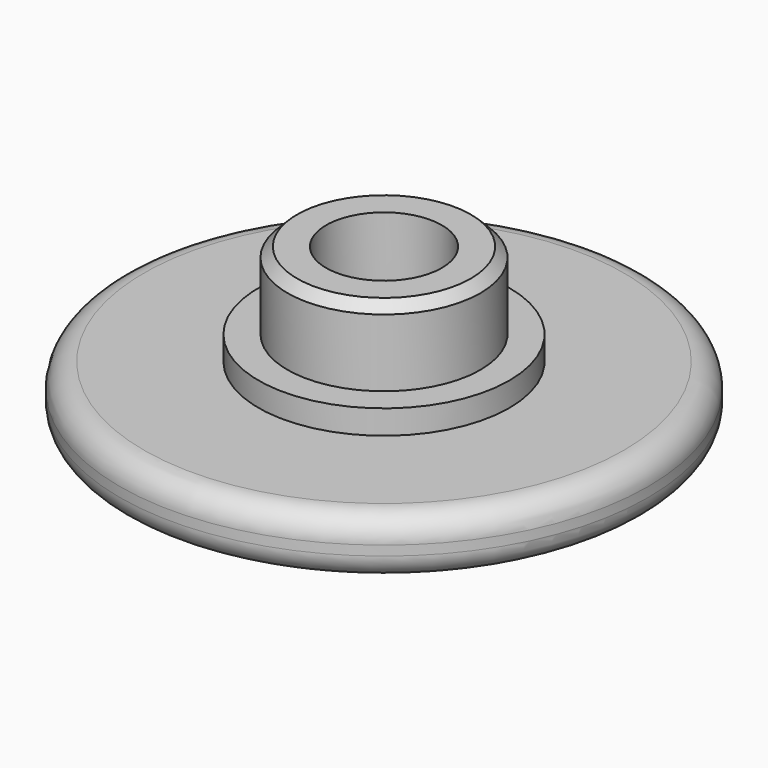
from build123d import *

# Parameters (mm, degrees)
F0_R      = 10.95
F1_DEPTH  = 2.4
F2_R      = 4
F3_DEPTH  = 4.2
F4_R      = 1
F5_R      = 5.2
F5_R_2    = 4
F6_DEPTH  = 1
F7_R      = 1
F8_R      = 8.5
F9_DEPTH  = 2
F11_SIZE  = 0.4
F12_R     = 3
F13_R     = 2.4
F14_DEPTH = 2.5


# Not quite as in the source:
# - a fillet or chamfer that OpenCascade refuses, or shapes differently, is made with other operations: its cross-section is extruded or revolved along the edge and cut away or added


with BuildPart() as f1:
    # F0 (on Top) → F1 (new body)
    with BuildSketch(Plane.XY):
        Circle(F0_R)
    extrude(amount=F1_DEPTH)

    # F2 (on face) → F3 (join)
    with BuildSketch(Plane.XY.offset(2.4)):
        Circle(F2_R)
    extrude(amount=F3_DEPTH)

    # F4
    f4_edges = [f1.edges().sort_by_distance(p)[0] for p in [
        (-10.95, 0, 2.4),
    ]]
    fillet(f4_edges, radius=F4_R)

    # F5 (on face) → F6 (join)
    with BuildSketch(Plane.XY.offset(2.4)):
        Circle(F5_R)
        Circle(F5_R_2, mode=Mode.SUBTRACT)
    extrude(amount=F6_DEPTH)

    # F7
    f7_edges = [f1.edges().sort_by_distance(p)[0] for p in [
        (-10.95, 0, 0),
    ]]
    fillet(f7_edges, radius=F7_R)

    # F8 (on face) → F9 (cut)
    with BuildSketch(Plane(origin=(0, 0, 0), x_dir=(1, 0, 0), z_dir=(0, 0, -1))):
        Circle(F8_R)
    extrude(amount=-F9_DEPTH, mode=Mode.SUBTRACT)

    # F10: fillet of radius 9 on 1 edges, made by hand

    # F10_s1 → F10_t2 (revolve)
    with BuildSketch(Plane.XZ):
        with BuildLine():
            ThreePointArc((8.5, 0), (5.8431457505, 1.4852813742), (2.8431457505, 2))
            Line((2.8431457505, 2), (8.5, 2))
            Line((8.5, 2), (8.5, 0))
        make_face()
    revolve(axis=Axis((0, 0, 2), (0, 0, -1)))

    # F11
    f11_edges = [f1.edges().sort_by_distance(p)[0] for p in [
        (-4, 0, 6.6),
    ]]
    chamfer(f11_edges, length=F11_SIZE)

    # F12
    f12_edges = [f1.edges().sort_by_distance(p)[0] for p in [
        (-8.5, 0, 0),
    ]]
    fillet(f12_edges, radius=F12_R)

    # F13 (on face) → F14 (cut)
    with BuildSketch(Plane.XY.offset(6.6)):
        Circle(F13_R)
    extrude(amount=-F14_DEPTH, mode=Mode.SUBTRACT)


solid = f1.part
